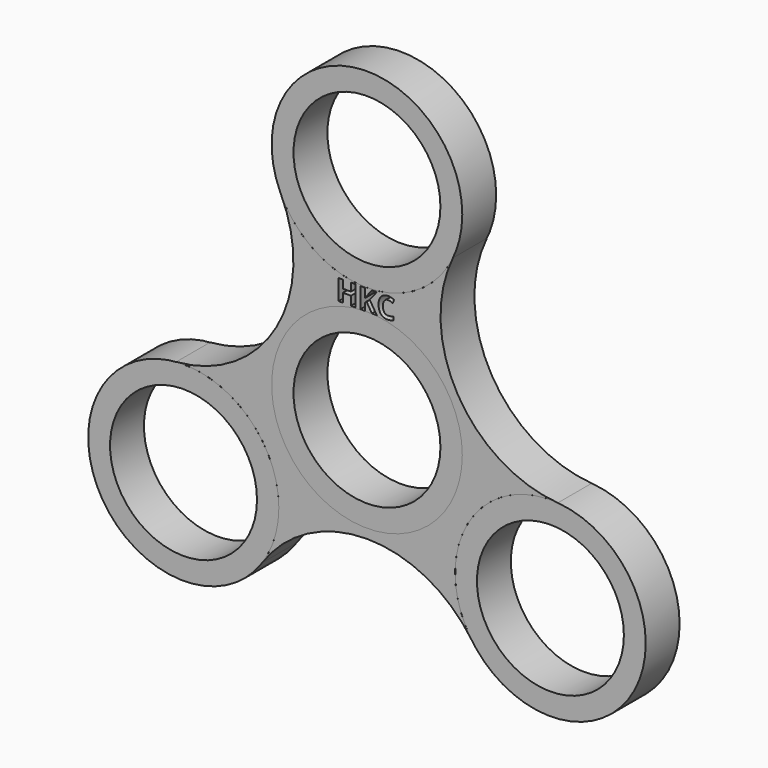
from build123d import *

# Parameters (mm, degrees)
F0_R         = 14.2875
F0_R_2       = 11.0109
F2_DEPTH     = 6.35
F1_R         = 14.2875
F3_TEXT_SIZE = 4.2903081824
F4_DEPTH     = 6.351


# Not quite as in the source:
# - a feature names something its author has since deleted; it is built from what else it names
# - Text() gives the source's letters only with a copy of the font that has no kerning and outlines rounded to 1/6400 em; it was checked with that copy


with BuildPart() as f2:
    # F0 (on Front) → F2 (new body)
    with BuildSketch(Plane.XZ):
        Circle(F0_R)
        Circle(F0_R_2, mode=Mode.SUBTRACT)
    extrude(amount=F2_DEPTH)


with BuildPart() as f2b:
    # F0 (on Front) → F2, piece 2 (new body)
    with BuildSketch(Plane.XZ):
        with Locations((0, 31.75)):
            Circle(F0_R)
        with Locations((0, 31.75)):
            Circle(F0_R_2, mode=Mode.SUBTRACT)
    extrude(amount=F2_DEPTH)


with BuildPart() as f2c:
    # F0 (on Front) → F2, piece 3 (new body)
    with BuildSketch(Plane.XZ):
        with Locations((27.4963065702, -15.875)):
            Circle(F0_R)
        with Locations((27.4963065702, -15.875)):
            Circle(F0_R_2, mode=Mode.SUBTRACT)
    extrude(amount=F2_DEPTH)


with BuildPart() as f2d:
    # F0 (on Front) → F2, piece 4 (new body)
    with BuildSketch(Plane.XZ):
        with Locations((-27.4963065702, -15.875)):
            Circle(F0_R)
        with Locations((-27.4963065702, -15.875)):
            Circle(F0_R_2, mode=Mode.SUBTRACT)
    extrude(amount=F2_DEPTH)


with BuildPart() as f2e:
    # F1 (on Front) → F2, piece 5 (new body)
    with BuildSketch(Plane.XZ):
        with BuildLine():
            ThreePointArc((12.8885060581, 25.584039585), (0, 17.4625), (-12.8885060581, 25.584039585))
            ThreePointArc((-12.8885060581, 25.584039585), (-13.5753968602, 7.8377590316), (-28.6006812411, -1.6302461293))
            ThreePointArc((-28.6006812411, -1.6302461293), (-17.7918255655, -5.3890234274), (-13.2088065702, -15.875))
            ThreePointArc((-13.2088065702, -15.875), (-13.8489912033, -20.103881593), (-15.7121751829, -23.9537934556))
            ThreePointArc((-15.7121751829, -23.9537934556), (0, -15.6755180632), (15.7121751829, -23.9537934556))
            ThreePointArc((15.7121751829, -23.9537934556), (15.1229686136, -8.73125), (28.6006812411, -1.6302461293))
            ThreePointArc((28.6006812411, -1.6302461293), (13.5753968602, 7.8377590316), (12.8885060581, 25.584039585))
        make_face()
        Circle(F1_R, mode=Mode.SUBTRACT)
    extrude(amount=F2_DEPTH)

    # F3 (on face) → F4 (cut, through all)
    with BuildSketch(Plane.XZ.offset(6.35)):
        with Locations((-4.6494889539, 14.2988404259)):
            Text('HKC', F3_TEXT_SIZE, font='Open Sans', font_style=FontStyle.BOLD, text_align=(TextAlign.LEFT, TextAlign.BOTTOM))
    extrude(amount=-F4_DEPTH, mode=Mode.SUBTRACT)


solid = Compound([f2.part, f2b.part, f2c.part, f2d.part, f2e.part])
